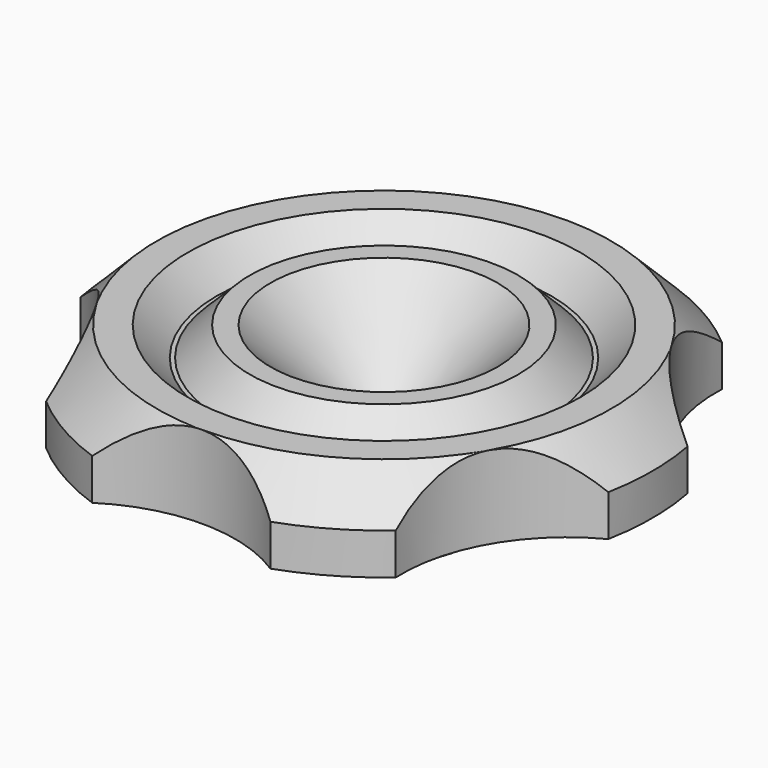
from build123d import *

# Parameters (mm, degrees)
F0_R             = 13
F1_DEPTH         = 4
F2_SIZE          = 2
F3_R             = 4.7
F4_DEPTH         = 4
F5_SIZE          = 0.5
F6_R             = 1.5
F7_DEPTH         = 25
F8_R             = 5.7
F8_R_2           = 4.7
F9_DEPTH         = 1.5
F10_R            = 8
F11_DEPTH        = 25
F11_COPIES_COUNT = 6
F12_R            = 9.5
F12_R_2          = 6.5
F13_DEPTH        = 1.4
F14_SIZE         = 1.39999
F15_SIZE         = 4


# Not quite as in the source:
# - a fillet or chamfer is up to 0.001 mm smaller than in the source, because OpenCascade refuses the exact size
# - a pattern or mirror of a feature is missing from the dataset's text; its kind, count and spacing are read off the source's solid


with BuildPart() as f1:
    # F0 (on Top) → F1 (new body)
    with BuildSketch(Plane.XY):
        Circle(F0_R)
    extrude(amount=F1_DEPTH)

    # F2
    f2_edges = [f1.edges().sort_by_distance(p)[0] for p in [
        (-13, 0, 4),
    ]]
    chamfer(f2_edges, length=F2_SIZE)

    # F3 (on face) → F4 (join)
    with BuildSketch(Plane(origin=(0, 0, 0), x_dir=(1, 0, 0), z_dir=(0, 0, -1))):
        Circle(F3_R)
    extrude(amount=F4_DEPTH)

    # F5
    f5_edges = [f1.edges().sort_by_distance(p)[0] for p in [
        (-4.7, 0, -4),
    ]]
    chamfer(f5_edges, length=F5_SIZE)

    # F6 (on face) → F7 (cut)
    with BuildSketch(Plane(origin=(0, 0, -4), x_dir=(1, 0, 0), z_dir=(0, 0, -1))):
        Circle(F6_R)
    extrude(amount=-F7_DEPTH, mode=Mode.SUBTRACT)

    # F8 (on face) → F9 (join)
    with BuildSketch(Plane(origin=(0, 0, 0), x_dir=(1, 0, 0), z_dir=(0, 0, -1))):
        Circle(F8_R)
        Circle(F8_R_2, mode=Mode.SUBTRACT)
    extrude(amount=F9_DEPTH)

    # F10 (on face) → F11 (cut)
    with BuildSketch(Plane(origin=(0, 0, 0), x_dir=(1, 0, 0), z_dir=(0, 0, -1))):
        with Locations((0, 19)):
            Circle(F10_R)
    f11 = extrude(amount=-F11_DEPTH, mode=Mode.SUBTRACT)

    # F11_copies: F11 ×6 about axis
    f11_copies_axis = Axis((0, 0, 0), (0, 0, 1))
    for i in range(1, F11_COPIES_COUNT):
        add(f11.rotate(f11_copies_axis, i * 360 / F11_COPIES_COUNT), mode=Mode.SUBTRACT)

    # F12 (on face) → F13 (cut)
    with BuildSketch(Plane.XY.offset(4)):
        Circle(F12_R)
        Circle(F12_R_2, mode=Mode.SUBTRACT)
    extrude(amount=-F13_DEPTH, mode=Mode.SUBTRACT)

    # F14 (size 1.4 in the source; OpenCascade refuses exactly that, so slightly less here)
    f14_edges = [f1.edges().sort_by_distance(p)[0] for p in [
        (-9.5, 0, 2.6),
        (-6.5, 0, 2.6),
    ]]
    chamfer(f14_edges, length=F14_SIZE)

    # F15
    f15_edges = [f1.edges().sort_by_distance(p)[0] for p in [
        (-1.5, 0, 4),
    ]]
    chamfer(f15_edges, length=F15_SIZE)


solid = f1.part
